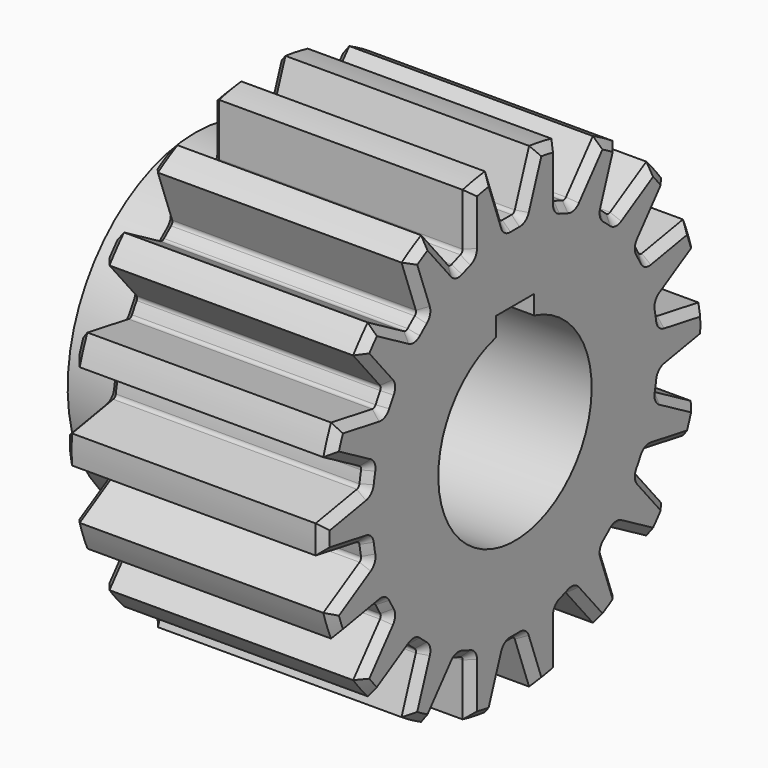
from build123d import *

# Parameters (mm, degrees)
F4_DEPTH        = 80.001
F4_COPIES_COUNT = 18
F5_R            = 1
F7_R            = 2
F8_SIZE         = 2
F9_R            = 24
F10_DEPTH       = 80.001
F2_W            = 12
F2_H            = 8
F11_DEPTH       = 80.001


# Not quite as in the source:
# - a feature of the source that left no trace in its solid (it failed there, or was rolled back) is left out
# - a pattern or mirror of a feature is missing from the dataset's text; its kind, count and spacing are read off the source's solid


with BuildPart() as f1:
    # F0 (on Front) → F1 (revolve)
    with BuildSketch(Plane.XZ):
        Polygon((-80, 40), (-80, 0), (0, 0), (0, 60), (-65, 60), (-65, 40), align=None)
    revolve(axis=Axis((-42.187795043, 0, 0), (-1, 0, 0)))

    # F3 (on face) → F4 (cut, through all)
    with BuildSketch(Plane.YZ):
        with BuildLine():
            ThreePointArc((-2.1835239212, 46.6088813778), (0, 46.66), (2.1835239212, 46.6088813778))
            Line((2.1835239212, 46.6088813778), (8.3158954322, 63.457433632))
            ThreePointArc((8.3158954322, 63.457433632), (0, 64), (-8.3158954322, 63.457433632))
            Line((-8.3158954322, 63.457433632), (-2.1835239212, 46.6088813778))
        make_face()
    f4 = extrude(amount=-F4_DEPTH, mode=Mode.SUBTRACT)

    # F4_copies: F4 ×18 about axis
    f4_copies_axis = Axis((0, 0, 0), (1, 0, 0))
    for i in range(1, F4_COPIES_COUNT):
        add(f4.rotate(f4_copies_axis, i * 360 / F4_COPIES_COUNT), mode=Mode.SUBTRACT)

    # F5
    f5_edges = [f1.edges().sort_by_distance(p)[0] for p in [
        (-32.5, 2.183524, 46.608881),
        (-32.5, -2.183524, 46.608881),
        (-32.5, -13.889335, 44.544831),
        (-32.5, -17.993018, 43.051213),
        (-32.5, -28.286935, 37.108017),
        (-32.5, -31.632288, 34.300932),
        (-32.5, -39.272713, 25.195428),
        (-32.5, -41.456237, 21.413454),
        (-32.5, -45.521623, 10.243899),
        (-32.5, -46.279953, 5.943196),
        (-32.5, -46.279953, -5.943196),
        (-32.5, -45.521623, -10.243899),
        (-32.5, -41.456237, -21.413454),
        (-32.5, -39.272713, -25.195428),
        (-32.5, -31.632288, -34.300932),
        (-32.5, -28.286935, -37.108017),
        (-32.5, -17.993018, -43.051213),
        (-32.5, -13.889335, -44.544831),
        (-32.5, -2.183524, -46.608881),
        (-32.5, 2.183524, -46.608881),
        (-32.5, 13.889335, -44.544831),
        (-32.5, 17.993018, -43.051213),
        (-32.5, 28.286935, -37.108017),
        (-32.5, 31.632288, -34.300932),
        (-32.5, 39.272713, -25.195428),
        (-32.5, 41.456237, -21.413454),
        (-32.5, 45.521623, -10.243899),
        (-32.5, 46.279953, -5.943196),
        (-32.5, 46.279953, 5.943196),
        (-32.5, 45.521623, 10.243899),
        (-32.5, 41.456237, 21.413454),
        (-32.5, 39.272713, 25.195428),
        (-32.5, 31.632288, 34.300932),
        (-32.5, 28.286935, 37.108017),
        (-32.5, 17.993018, 43.051213),
        (-32.5, 13.889335, 44.544831),
    ]]
    fillet(f5_edges, radius=F5_R)

    # F7
    f7_edges = [f1.edges().sort_by_distance(p)[0] for p in [
        (-65, 0, -40),
    ]]
    fillet(f7_edges, radius=F7_R)

    # F8
    f8_edges = [f1.edges().sort_by_distance(p)[0] for p in [
        (-65, 0, -42),
        (-65, 4.672597, 53.447552),
        (-65, 2.054075, 46.808558),
        (-65, 10.418891, 59.088465),
        (-65, 0, 46.66),
        (-65, 13.889335, 51.822393),
        (-65, -2.054075, 46.808558),
        (-65, 14.079271, 44.688191),
        (-65, -4.672597, 53.447552),
        (-65, 15.95866, 43.846058),
        (-65, -10.418891, 59.088465),
        (-65, 17.939668, 43.283121),
        (-65, -13.889335, 51.822393),
        (-65, 22.670944, 48.626148),
        (-65, -14.079271, 44.688191),
        (-65, 30, 51.961524),
        (-65, -15.95866, 43.846058),
        (-65, 30.776008, 43.946688),
        (-65, -17.939668, 43.283121),
        (-65, 28.514449, 37.177769),
        (-65, -22.670944, 48.626148),
        (-65, 29.99247, 35.743634),
        (-65, -30, 51.961524),
        (-65, 31.661473, 34.537102),
        (-65, -30.776008, 43.946688),
        (-65, 37.934841, 37.939713),
        (-65, -28.514449, 37.177769),
        (-65, 45.962667, 38.567257),
        (-65, -29.99247, 35.743634),
        (-65, 43.95064, 30.770363),
        (-65, -31.661473, 34.537102),
        (-65, 39.510363, 25.18316),
        (-65, -37.934841, 37.939713),
        (-65, 40.408745, 23.33),
        (-65, -45.962667, 38.567257),
        (-65, 41.564437, 21.625398),
        (-65, -43.95064, 30.770363),
        (-65, 48.623236, 22.677189),
        (-65, -39.510363, 25.18316),
        (-65, 56.381557, 20.521209),
        (-65, -40.408745, 23.33),
        (-65, 51.824176, 13.882679),
        (-65, -41.564437, 21.625398),
        (-65, 45.740744, 10.151089),
        (-65, -48.623236, 22.677189),
        (-65, 45.95113, 8.102424),
        (-65, -56.381557, 20.521209),
        (-65, 46.454117, 6.105352),
        (-65, -51.824176, 13.882679),
        (-65, 53.446952, 4.679461),
        (-65, -45.740744, 10.151089),
        (-65, 60, 0),
        (-65, -45.95113, 8.102424),
        (-65, 53.446952, -4.679461),
        (-65, -46.454117, 6.105352),
        (-65, 46.454117, -6.105352),
        (-65, -53.446952, 4.679461),
        (-65, 45.95113, -8.102424),
        (-65, -60, 0),
        (-65, 45.740744, -10.151089),
        (-65, -53.446952, -4.679461),
        (-65, 51.824176, -13.882679),
        (-65, -46.454117, -6.105352),
        (-65, 56.381557, -20.521209),
        (-65, -45.95113, -8.102424),
        (-65, 48.623236, -22.677189),
        (-65, -45.740744, -10.151089),
        (-65, 41.564437, -21.625398),
        (-65, -51.824176, -13.882679),
        (-65, 40.408745, -23.33),
        (-65, -56.381557, -20.521209),
        (-65, 39.510363, -25.18316),
        (-65, -48.623236, -22.677189),
        (-65, 43.95064, -30.770363),
        (-65, -41.564437, -21.625398),
        (-65, 45.962667, -38.567257),
        (-65, -40.408745, -23.33),
        (-65, 37.934841, -37.939713),
        (-65, -39.510363, -25.18316),
        (-65, 31.661473, -34.537102),
        (-65, -43.95064, -30.770363),
        (-65, 29.99247, -35.743634),
        (-65, -45.962667, -38.567257),
        (-65, 28.514449, -37.177769),
        (-65, -37.934841, -37.939713),
        (-65, 30.776008, -43.946688),
        (-65, -31.661473, -34.537102),
        (-65, 30, -51.961524),
        (-65, -29.99247, -35.743634),
        (-65, 22.670944, -48.626148),
        (-65, -28.514449, -37.177769),
        (-65, 17.939668, -43.283121),
        (-65, -30.776008, -43.946688),
        (-65, 15.95866, -43.846058),
        (-65, -30, -51.961524),
        (-65, 14.079271, -44.688191),
        (-65, -22.670944, -48.626148),
        (-65, 13.889335, -51.822393),
        (-65, -17.939668, -43.283121),
        (-65, 10.418891, -59.088465),
        (-65, -15.95866, -43.846058),
        (-65, 4.672597, -53.447552),
        (-65, -14.079271, -44.688191),
        (-65, 2.054075, -46.808558),
        (-65, -13.889335, -51.822393),
        (-65, 0, -46.66),
        (-65, -10.418891, -59.088465),
        (-65, -2.054075, -46.808558),
        (-65, -4.672597, -53.447552),
        (0, 13.889335, 51.822393),
        (0, 14.079271, 44.688191),
        (0, 10.418891, 59.088465),
        (0, 15.95866, 43.846058),
        (0, 4.672597, 53.447552),
        (0, 17.939668, 43.283121),
        (0, 2.054075, 46.808558),
        (0, 22.670944, 48.626148),
        (0, 0, 46.66),
        (0, 30, 51.961524),
        (0, -2.054075, 46.808558),
        (0, 30.776008, 43.946688),
        (0, -4.672597, 53.447552),
        (0, 28.514449, 37.177769),
        (0, -10.418891, 59.088465),
        (0, 29.99247, 35.743634),
        (0, -13.889335, 51.822393),
        (0, 31.661473, 34.537102),
        (0, -14.079271, 44.688191),
        (0, 37.934841, 37.939713),
        (0, -15.95866, 43.846058),
        (0, 45.962667, 38.567257),
        (0, -17.939668, 43.283121),
        (0, 43.95064, 30.770363),
        (0, -22.670944, 48.626148),
        (0, 39.510363, 25.18316),
        (0, -30, 51.961524),
        (0, 40.408745, 23.33),
        (0, -30.776008, 43.946688),
        (0, 41.564437, 21.625398),
        (0, -28.514449, 37.177769),
        (0, 48.623236, 22.677189),
        (0, -29.99247, 35.743634),
        (0, 56.381557, 20.521209),
        (0, -31.661473, 34.537102),
        (0, 51.824176, 13.882679),
        (0, -37.934841, 37.939713),
        (0, 45.740744, 10.151089),
        (0, -45.962667, 38.567257),
        (0, 45.95113, 8.102424),
        (0, -43.95064, 30.770363),
        (0, 46.454117, 6.105352),
        (0, -39.510363, 25.18316),
        (0, 53.446952, 4.679461),
        (0, -40.408745, 23.33),
        (0, 60, 0),
        (0, -41.564437, 21.625398),
        (0, 53.446952, -4.679461),
        (0, -48.623236, 22.677189),
        (0, 46.454117, -6.105352),
        (0, -56.381557, 20.521209),
        (0, 45.95113, -8.102424),
        (0, -51.824176, 13.882679),
        (0, 45.740744, -10.151089),
        (0, -45.740744, 10.151089),
        (0, 51.824176, -13.882679),
        (0, -45.95113, 8.102424),
        (0, 56.381557, -20.521209),
        (0, -46.454117, 6.105352),
        (0, 48.623236, -22.677189),
        (0, -53.446952, 4.679461),
        (0, 41.564437, -21.625398),
        (0, -60, 0),
        (0, 40.408745, -23.33),
        (0, -53.446952, -4.679461),
        (0, 39.510363, -25.18316),
        (0, -46.454117, -6.105352),
        (0, 43.95064, -30.770363),
        (0, -45.95113, -8.102424),
        (0, 45.962667, -38.567257),
        (0, -45.740744, -10.151089),
        (0, 37.934841, -37.939713),
        (0, -51.824176, -13.882679),
        (0, 31.661473, -34.537102),
        (0, -56.381557, -20.521209),
        (0, 29.99247, -35.743634),
        (0, -48.623236, -22.677189),
        (0, 28.514449, -37.177769),
        (0, -41.564437, -21.625398),
        (0, 30.776008, -43.946688),
        (0, -40.408745, -23.33),
        (0, 30, -51.961524),
        (0, -39.510363, -25.18316),
        (0, 22.670944, -48.626148),
        (0, -43.95064, -30.770363),
        (0, 17.939668, -43.283121),
        (0, -45.962667, -38.567257),
        (0, 15.95866, -43.846058),
        (0, -37.934841, -37.939713),
        (0, 14.079271, -44.688191),
        (0, -31.661473, -34.537102),
        (0, 13.889335, -51.822393),
        (0, -29.99247, -35.743634),
        (0, 10.418891, -59.088465),
        (0, -28.514449, -37.177769),
        (0, 4.672597, -53.447552),
        (0, -30.776008, -43.946688),
        (0, 2.054075, -46.808558),
        (0, -30, -51.961524),
        (0, 0, -46.66),
        (0, -22.670944, -48.626148),
        (0, -2.054075, -46.808558),
        (0, -17.939668, -43.283121),
        (0, -4.672597, -53.447552),
        (0, -15.95866, -43.846058),
        (0, -10.418891, -59.088465),
        (0, -14.079271, -44.688191),
        (0, -13.889335, -51.822393),
    ]]
    chamfer(f8_edges, length=F8_SIZE)

    # F9 (on face) → F10 (cut, through all)
    with BuildSketch(Plane.YZ):
        Circle(F9_R)
    extrude(amount=-F10_DEPTH, mode=Mode.SUBTRACT)

    # F2 (on face) → F11 (cut, through all)
    with BuildSketch(Plane.YZ):
        with Locations((0, 24)):
            Rectangle(F2_W, F2_H)
    extrude(amount=-F11_DEPTH, mode=Mode.SUBTRACT)


solid = f1.part
